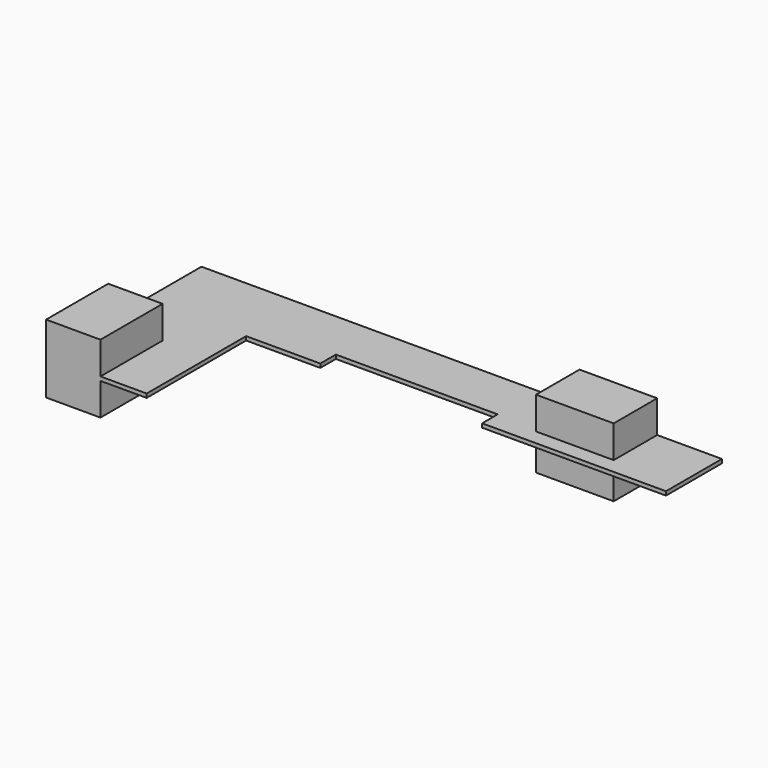
from build123d import *

# Parameters (mm, degrees)
F1_DEPTH = 1.5
F2_W     = 42
F2_H     = 25
F3_DEPTH = 60
F5_W     = 42
F5_H     = 25
F6_DEPTH = 60
F7_W     = 125
F7_H     = 15
F8_DEPTH = 25


# Not quite as in the source:
# - a pattern or mirror of a feature is missing from the dataset's text; its kind, count and spacing are read off the source's solid


with BuildPart() as f1:
    # F0 (on Top) → F1 (new body, symmetric)
    with BuildSketch(Plane.XY):
        Polygon((-77.7, -96), (0, -96), (0, 0), (324.3, 0), (324.3, 54), (-77.7, 54), align=None)
    extrude(amount=F1_DEPTH, both=True)

    # F2 (on face) → F3 (join)
    with BuildSketch(Plane.XZ.offset(96)):
        with Locations((-56.7, -14)):
            Rectangle(F2_W, F2_H)
    f3 = extrude(amount=-F3_DEPTH)

    # F3_copies: F3 across plane
    add(f3.mirror(Plane.XY))

    # F5 (on offset) → F6 (join)
    with BuildSketch(Plane.YZ.offset(274.3)):
        with Locations((33, -14)):
            Rectangle(F5_W, F5_H)
    f6 = extrude(amount=-F6_DEPTH)

    # F6_copies: F6 across plane
    add(f6.mirror(Plane.XY))

    # F7 (on face) → F8 (cut)
    with BuildSketch(Plane.XY.offset(1.5)):
        with Locations((119.8, 7.5)):
            Rectangle(F7_W, F7_H)
    extrude(amount=-F8_DEPTH, mode=Mode.SUBTRACT)


solid = f1.part
